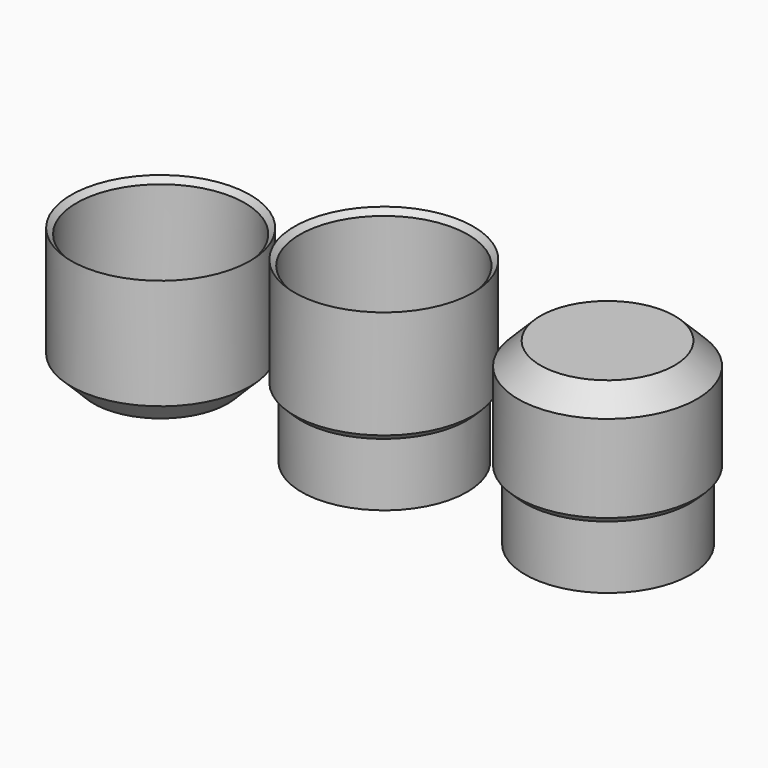
from build123d import *

# Parameters (mm, degrees)
F0_R          = 20
F1_DEPTH      = 30
F0_R_2        = 18.5
F0_R_3        = 10
F2_DEPTH      = 15
F3_R          = 20
F4_DEPTH      = 25
F4_DEPTH_BACK = 1
F3_R_2        = 18.5
F5_T          = -1.2
F5_2_T        = -1.2
F5_3_T        = -1.2
F6_DEPTH      = 25.0000003725
F7_3_S7_R     = 17.3
F7_3_T8_DEPTH = 28
F8_2_S5_R     = 18.5
F8_2_T6_DEPTH = 30
F8_3_S5_R     = 18.5
F8_3_T6_DEPTH = 30
F9_SIZE       = 5
F9_2_SIZE     = 5


# Not quite as in the source:
# - a fillet or chamfer that OpenCascade refuses, or shapes differently, is made with other operations: its cross-section is extruded or revolved along the edge and cut away or added


with BuildPart() as f1:
    # F0 (on Top) → F1 (new body)
    with BuildSketch(Plane.XY):
        with Locations((-49.8913675547, 0)):
            Circle(F0_R)
    extrude(amount=F1_DEPTH)

    # F5
    f5_openings = [f1.faces().sort_by_distance(p)[0] for p in [
        (-49.891368, 0, 30),
    ]]
    offset(amount=F5_T, openings=f5_openings)

    # F7: chamfer of 7 on 1 edges, made by hand

    # F7_s1 → F7_t2 (revolve)
    with BuildSketch(Plane.XZ):
        Polygon((-31.0913675547, 8.2), (-38.0913675547, 1.2), (-31.0913675547, 1.2), align=None)
    revolve(axis=Axis((-49.8913675547, 0, 1.2), (0, 0, -1)))

    # F8: chamfer of 1.5 on 1 edges, made by hand

    # F8_s1 → F8_t2 (revolve, cut)
    with BuildSketch(Plane.XZ):
        Polygon((-29.5913675547, 30), (-31.0913675547, 28.5), (-31.0913675547, 30), align=None)
    revolve(axis=Axis((-49.8913675547, 0, 30), (0, 0, 1)), mode=Mode.SUBTRACT)

    # F9
    f9_edges = [f1.edges().sort_by_distance(p)[0] for p in [
        (-69.891368, 0, 0),
    ]]
    chamfer(f9_edges, length=F9_SIZE)


with BuildPart() as f2:
    # F0 (on Top) → F2 (new body)
    with BuildSketch(Plane.XY):
        with Locations((0.1086324453, 0)):
            Circle(F0_R_2)
        with Locations((0.1086324453, 0)):
            Circle(F0_R_3, mode=Mode.SUBTRACT)
        with Locations((0.1086324453, 0)):
            Circle(F0_R_3)
    extrude(amount=F2_DEPTH)

    # F3 (on face) → F4, piece 2 (join, two sides)
    with BuildSketch(Plane.XY.offset(15)) as f4_2_sk:
        Circle(F3_R)
        with Locations((0.1086324453, 0)):
            Circle(F3_R_2, mode=Mode.SUBTRACT)
        with Locations((0.1086324453, 0)):
            Circle(F3_R_2)
    extrude(amount=F4_DEPTH)
    extrude(f4_2_sk.sketch, amount=-F4_DEPTH_BACK)

    # F5#2
    f5_2_openings = [f2.faces().sort_by_distance(p)[0] for p in [
        (0, 0, 40),
    ]]
    offset(amount=F5_2_T, openings=f5_2_openings, kind=Kind.INTERSECTION)

    # F0 (on Top) → F6 (cut)
    with BuildSketch(Plane.XY):
        with Locations((0.1086324453, 0)):
            Circle(F0_R_3)
    extrude(amount=F6_DEPTH, mode=Mode.SUBTRACT)

    # F7#2: chamfer of 7 on 2 edges, made by hand

    # F7_2_s1 → F7_2_t2 (revolve)
    with BuildSketch(Plane.XZ):
        Polygon((10.4086324453, 1.2), (17.4086324453, 8.2), (17.4086324453, 1.2), align=None)
    revolve(axis=Axis((0.1086324453, 0, 1.2), (0, 0, -1)))

    # F8#2: chamfer of 1.5 on 2 edges, made by hand


with BuildPart() as f2b:
    # F0 (on Top) → F2, piece 2 (new body)
    with BuildSketch(Plane.XY):
        with Locations((50.1086324453, 0)):
            Circle(F0_R_2)
    extrude(amount=F2_DEPTH)

    # F3 (on face) → F4 (join, two sides)
    with BuildSketch(Plane.XY.offset(15)) as f4_sk:
        with Locations((50, 0)):
            Circle(F3_R)
    extrude(amount=F4_DEPTH)
    extrude(f4_sk.sketch, amount=-F4_DEPTH_BACK)

    # F5#3
    f5_3_openings = [f2b.faces().sort_by_distance(p)[0] for p in [
        (50.108632, 0, 0),
    ]]
    offset(amount=F5_3_T, openings=f5_3_openings, kind=Kind.INTERSECTION)

    # F7#3: chamfer of 7 on 3 edges, made by hand

    # F7_3_s1 → F7_3_t2 (revolve)
    with BuildSketch(Plane.XZ):
        Polygon((68.8, 31.8), (61.8, 38.8), (68.8, 38.8), align=None)
    revolve(axis=Axis((50, 0, 38.8), (0, 0, 1)))


with BuildPart() as f7_3_tool4:
    # F7_3_s5 → F7_3_t6 (revolve)
    with BuildSketch(Plane.XZ):
        Polygon((61.8, 15.2), (68.8, 22.2), (68.8, 15.2), align=None)
    revolve(axis=Axis((50, 0, 15.2), (0, 0, 1)))

    # F7_3_s7 → F7_3_t8 (cut, symmetric)
    with BuildSketch(Plane.XY.offset(18.7)):
        with Locations((50.1086324453, 0)):
            Circle(F7_3_S7_R)
    extrude(amount=F7_3_T8_DEPTH, both=True, mode=Mode.SUBTRACT)


with BuildPart() as f2b_1:
    add(f2b.part)

    # F7_3_t3: union F7_3_tool4
    add(f7_3_tool4.part)

    # F8#3: chamfer of 1.5 on 1 edges, made by hand


with BuildPart() as f8_2_tool2:
    # F8_2_s3 → F8_2_t4 (revolve)
    with BuildSketch(Plane.XZ):
        Polygon((18.5, 14), (20, 15.5), (20, 14), align=None)
    revolve(axis=Axis((0, 0, 14), (0, 0, 1)))

    # F8_2_s5 → F8_2_t6 (cut, symmetric)
    with BuildSketch(Plane.XY.offset(14.8)):
        with Locations((0.1086324453, 0)):
            Circle(F8_2_S5_R)
    extrude(amount=F8_2_T6_DEPTH, both=True, mode=Mode.SUBTRACT)


with BuildPart() as f2_1:
    add(f2.part)

    # F8_2_t1: cut F8_2_tool2
    add(f8_2_tool2.part, mode=Mode.SUBTRACT)

    # F8_2_s7 → F8_2_t8 (revolve, cut)
    with BuildSketch(Plane.XZ):
        Polygon((20.3, 40), (18.8, 38.5), (18.8, 40), align=None)
    revolve(axis=Axis((0, 0, 40), (0, 0, 1)), mode=Mode.SUBTRACT)


with BuildPart() as f8_3_tool2:
    # F8_3_s3 → F8_3_t4 (revolve)
    with BuildSketch(Plane.XZ):
        Polygon((68.5, 14), (70, 15.5), (70, 14), align=None)
    revolve(axis=Axis((50, 0, 14), (0, 0, 1)))

    # F8_3_s5 → F8_3_t6 (cut, symmetric)
    with BuildSketch(Plane.XY.offset(14.8)):
        with Locations((50.1086324453, 0)):
            Circle(F8_3_S5_R)
    extrude(amount=F8_3_T6_DEPTH, both=True, mode=Mode.SUBTRACT)


with BuildPart() as f2b_2:
    add(f2b_1.part)

    # F8_3_t1: cut F8_3_tool2
    add(f8_3_tool2.part, mode=Mode.SUBTRACT)

    # F9#2
    f9_2_edges = [f2b_2.edges().sort_by_distance(p)[0] for p in [
        (30, 0, 40),
    ]]
    chamfer(f9_2_edges, length=F9_2_SIZE)


solid = Compound([f1.part, f2_1.part, f2b_2.part])
